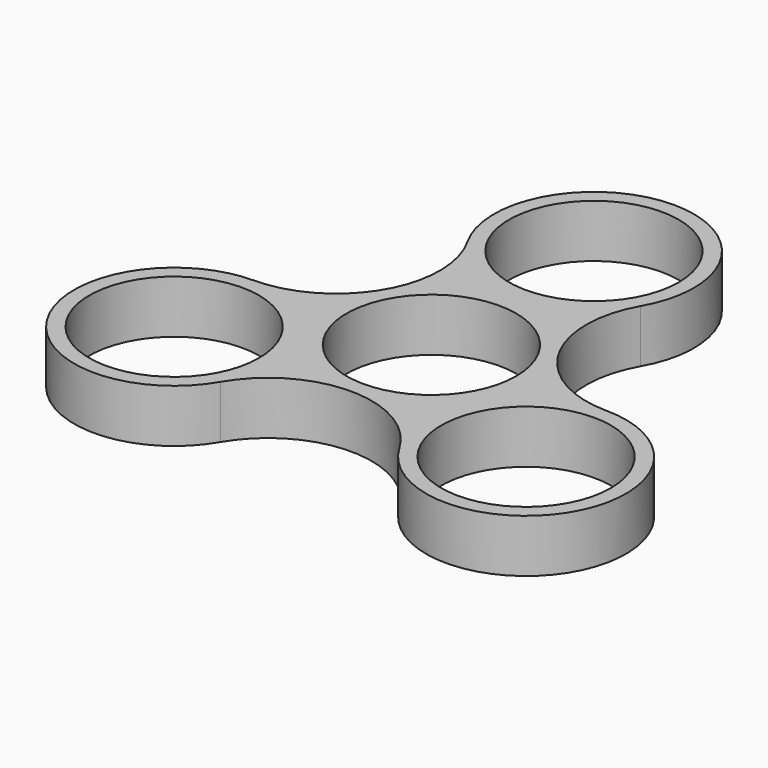
from build123d import *

# Parameters (mm, degrees)
F0_R     = 11.2
F1_DEPTH = 7


# Not quite as in the source:
# - ends of sketch curves that miss each other by under 0.0002 mm in the source are joined


with BuildPart() as f1:
    # F0 (on Top) → F1 (new body)
    with BuildSketch(Plane.XY):
        with BuildLine():
            ThreePointArc((23.1851437087, -0.209827322), (11.4809905002, 6.6524743947), (11.4315817283, 20.219933477))
            ThreePointArc((11.4315817283, 20.219933477), (-9.27972e-05, 40.0198531118), (-11.4314889311, 20.2197727475))
            ThreePointArc((-11.4314889311, 20.2197727475), (-11.4807071504, 6.6523126094), (-23.1847645, -0.2101533167))
            ThreePointArc((-23.1847645, -0.2101533167), (-29.8083976457, -1.9681833019), (-34.6579717698, -6.8101680492))
            ThreePointArc((-34.6579717698, -6.8101680492), (-29.8265597829, -24.8415250126), (-11.7950971191, -20.0105075285))
            ThreePointArc((-11.7950971191, -20.0105075285), (0.0002818311, -13.2693854266), (11.7957555615, -20.0103416826))
            ThreePointArc((11.7957555615, -20.0103416826), (29.8270373152, -24.8412493105), (34.6587334242, -6.8101809544))
            ThreePointArc((34.6587334242, -6.8101809544), (29.8271641282, -1.97867959), (23.2271516953, -0.2102613183))
            ThreePointArc((23.2271516953, -0.2102613183), (23.2061475356, -0.2100604335), (23.1851437087, -0.209827322))
        make_face()
        with Locations((-23.2263900417, -13.4100876845)):
            Circle(F0_R, mode=Mode.SUBTRACT)
        Circle(F0_R, mode=Mode.SUBTRACT)
        with Locations((23.2269557018, -13.4097611005)):
            Circle(F0_R, mode=Mode.SUBTRACT)
        with Locations((0, 26.8198531121)):
            Circle(F0_R, mode=Mode.SUBTRACT)
        with BuildLine():
            ThreePointArc((34.6587334242, -6.8101809544), (29.8090523926, -1.967907966), (23.1851437087, -0.209827322))
            ThreePointArc((23.1851437087, -0.209827322), (23.2061475356, -0.2100604335), (23.2271516953, -0.2102613183))
            ThreePointArc((23.2271516953, -0.2102613183), (29.8271641282, -1.97867959), (34.6587334242, -6.8101809544))
        make_face()
        with BuildLine():
            ThreePointArc((11.7957555615, -20.0103416826), (29.8273248567, -24.8417502494), (34.6587334242, -6.8101809544))
            ThreePointArc((34.6587334242, -6.8101809544), (29.8270373152, -24.8412493105), (11.7957555615, -20.0103416826))
        make_face()
        with BuildLine():
            ThreePointArc((-11.7950971191, -20.0105075285), (-29.8265597829, -24.8415250126), (-34.6579717698, -6.8101680492))
            ThreePointArc((-34.6579717698, -6.8101680492), (-29.8268485886, -24.8420252216), (-11.7950971191, -20.0105075285))
        make_face()
    extrude(amount=F1_DEPTH)


solid = f1.part
